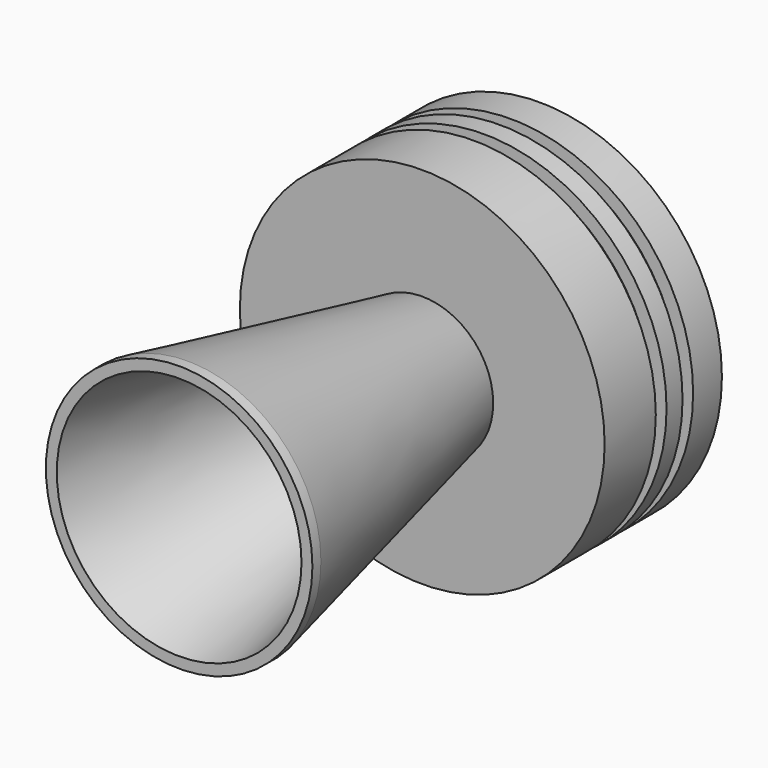
from build123d import *

# Parameters (mm, degrees)
F0_R      = 25.4
F0_R_2    = 7.9375
F1_DEPTH  = 57.912
F2_SIZE2  = 11.8776606661
F2_SIZE   = 55.88
F3_R      = 34.7599
F3_R_2    = 13.5223393339
F3_R_3    = 7.9375
F4_DEPTH  = 12.192
F6_R      = 32.2199
F6_R_2    = 8.4234043
F7_DEPTH  = 2.54
F8_R      = 34.7754798106
F8_R_2    = 32.2199
F8_R_3    = 8.4234043
F9_DEPTH  = 3.81
F10_R     = 32.2199
F10_R_2   = 8.4234043
F11_DEPTH = 2.54
F13_R     = 34.7599
F13_R_2   = 32.2199
F12_R     = 32.2199
F12_R_2   = 8.4234043
F14_DEPTH = 6.858
F15_SIZE2 = 14.6646968374
F15_SIZE  = 25.4


# Not quite as in the source:
# - a fillet or chamfer that OpenCascade refuses, or shapes differently, is made with other operations: its cross-section is extruded or revolved along the edge and cut away or added


with BuildPart() as f1:
    # F0 (on Front) → F1 (new body)
    with BuildSketch(Plane.XZ):
        Circle(F0_R)
        Circle(F0_R_2, mode=Mode.SUBTRACT)
    extrude(amount=F1_DEPTH)

    # F2
    f2_edges = [f1.edges().sort_by_distance(p)[0] for p in [
        (-25.4, 0, 0),
    ]]
    f2_side = f1.faces().sort_by_distance((-25.4, -28.956, 0))[0]
    chamfer(f2_edges, length=F2_SIZE, length2=F2_SIZE2, reference=f2_side)

    # F3 (on face) → F4 (join)
    with BuildSketch(Plane(origin=(0, 0, 0), x_dir=(-1, 0, 0), z_dir=(0, 1, 0))):
        Circle(F3_R)
        Circle(F3_R_2, mode=Mode.SUBTRACT)
        Circle(F3_R_2)
        Circle(F3_R_3, mode=Mode.SUBTRACT)
    extrude(amount=F4_DEPTH)

    # F5: chamfer of 72.39 x 15.3869694993 on 1 edges, made by hand

    # F5_s1 → F5_t2 (revolve, cut)
    with BuildSketch(Plane.XY):
        Polygon((23.3244694993, -57.912), (7.9375, 14.478), (7.9375, -57.912), align=None)
    revolve(axis=Axis((0, -57.912, 0), (0, -1, 0)), mode=Mode.SUBTRACT)

    # F6 (on face) → F7 (join)
    with BuildSketch(Plane(origin=(0, 12.192, 0), x_dir=(-1, 0, 0), z_dir=(0, 1, 0))):
        Circle(F6_R)
        Circle(F6_R_2, mode=Mode.SUBTRACT)
    extrude(amount=F7_DEPTH)

    # F8 (on face) → F9 (join)
    with BuildSketch(Plane(origin=(0, 14.732, 0), x_dir=(-1, 0, 0), z_dir=(0, 1, 0))):
        Circle(F8_R)
        Circle(F8_R_2, mode=Mode.SUBTRACT)
        Circle(F8_R_2)
        Circle(F8_R_3, mode=Mode.SUBTRACT)
    extrude(amount=F9_DEPTH)

    # F10 (on face) → F11 (join)
    with BuildSketch(Plane(origin=(0, 18.542, 0), x_dir=(-1, 0, 0), z_dir=(0, 1, 0))):
        Circle(F10_R)
        Circle(F10_R_2, mode=Mode.SUBTRACT)
    extrude(amount=F11_DEPTH)

    # F13 (on face) + F12 (on face) → F14 (join)
    with BuildSketch(Plane(origin=(0, 21.082, 0), x_dir=(-1, 0, 0), z_dir=(0, 1, 0))):
        Circle(F13_R)
        Circle(F13_R_2, mode=Mode.SUBTRACT)
    with BuildSketch(Plane(origin=(0, 21.082, 0), x_dir=(-1, 0, 0), z_dir=(0, 1, 0))):
        Circle(F12_R)
        Circle(F12_R_2, mode=Mode.SUBTRACT)
    extrude(amount=F14_DEPTH)

    # F15
    f15_edges = [f1.edges().sort_by_distance(p)[0] for p in [
        (8.423404, 27.94, 0),
    ]]
    f15_side = f1.faces().sort_by_distance((33.776742, 27.94, 0))[0]
    chamfer(f15_edges, length=F15_SIZE, length2=F15_SIZE2, reference=f15_side)


solid = f1.part
